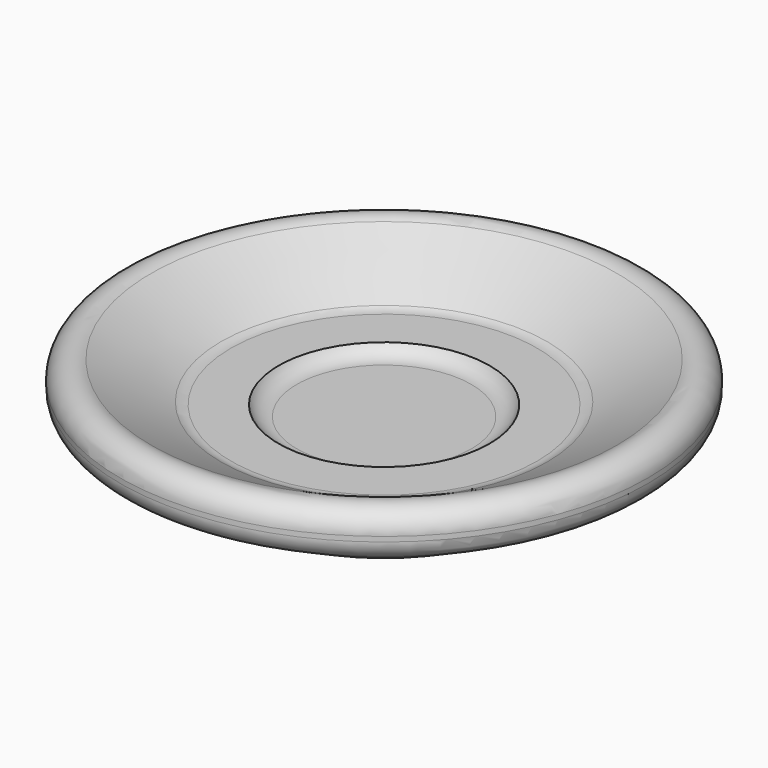
from build123d import *

# Parameters (mm, degrees)
F3_R     = 25.4
F4_DEPTH = 2.54


# Not quite as in the source:
# - a fillet or chamfer that OpenCascade refuses, or shapes differently, is made with other operations: its cross-section is extruded or revolved along the edge and cut away or added


with BuildPart() as f2:
    # F0 (on Front) → F2 (revolve)
    with BuildSketch(Plane.XZ):
        Polygon((63.5, 13.6071443505), (63.5, 26.3071443505), (38.1, 12.7), (0, 12.7), (0, 0), (38.1, 0), align=None)
    revolve(axis=Axis((0, 0, 37.3074896634), (0, 0, 1)))

    # F3 (on face) → F4 (cut)
    with BuildSketch(Plane.XY.offset(12.7)):
        Circle(F3_R)
    extrude(amount=-F4_DEPTH, mode=Mode.SUBTRACT)

    # F5: fillet of radius 5.08 on 4 edges, made by hand

    # F5_s1 → F5_t2 (revolve)
    with BuildSketch(Plane.XZ):
        with BuildLine():
            ThreePointArc((39.2238860188, 13.3020818618), (38.0616448552, 12.8528190544), (36.8250010386, 12.7))
            Line((36.8250010386, 12.7), (38.1, 12.7))
            Line((38.1, 12.7), (39.2238860188, 13.3020818618))
        make_face()
    revolve(axis=Axis((0, 0, 12.7), (0, 0, 1)))

    # F5_s3 → F5_t4 (revolve)
    with BuildSketch(Plane.XZ):
        with BuildLine():
            ThreePointArc((25.4, 12.7), (23.5405909488, 10.8405909488), (21.0005909488, 10.16))
            Line((21.0005909488, 10.16), (25.4, 10.16))
            Line((25.4, 10.16), (25.4, 12.7))
        make_face()
    revolve(axis=Axis((0, 0, 10.16), (0, 0, 1)))

    # F5_s5 → F5_t6 (revolve, cut)
    with BuildSketch(Plane.XZ):
        with BuildLine():
            ThreePointArc((56.0211150199, 22.3005983857), (61.0296038302, 22.181162535), (63.5, 17.8226802476))
            Line((63.5, 17.8226802476), (63.5, 26.3071443505))
            Line((63.5, 26.3071443505), (56.0211150199, 22.3005983857))
        make_face()
    revolve(axis=Axis((0, 0, 26.3071443505), (0, 0, 1)), mode=Mode.SUBTRACT)

    # F5_s7 → F5_t8 (revolve, cut)
    with BuildSketch(Plane.XZ):
        with BuildLine():
            ThreePointArc((63.5, 16.6487507133), (62.7784822874, 14.0391468831), (60.8188849801, 12.1708325751))
            Line((60.8188849801, 12.1708325751), (63.5, 13.6071443505))
            Line((63.5, 13.6071443505), (63.5, 16.6487507133))
        make_face()
    revolve(axis=Axis((0, 0, 13.6071443505), (0, 0, 1)), mode=Mode.SUBTRACT)


solid = f2.part
